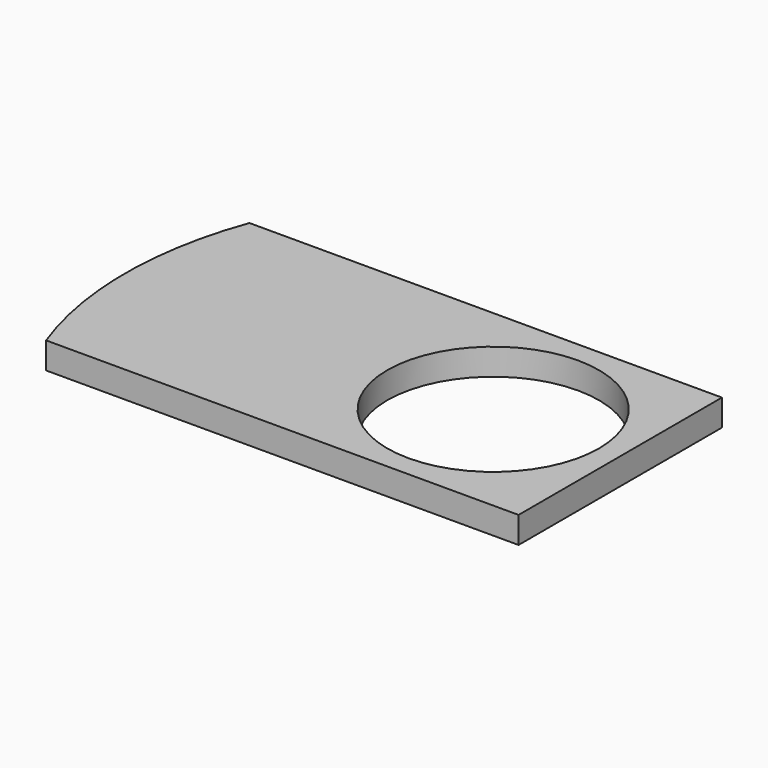
from build123d import *

# Parameters (mm, degrees)
F0_R     = 2
F1_DEPTH = 0.5


with BuildPart() as f1:
    # F0 (on Top) → F1 (new body)
    with BuildSketch(Plane.XY):
        with BuildLine():
            Line((-5.986860613, 2.4), (-6.5224611919, 2.4))
            ThreePointArc((-6.5224611919, 2.4), (-6.95, 0), (-6.5224611919, -2.4))
            Line((-6.5224611919, -2.4), (-5.986860613, -2.4))
            ThreePointArc((-5.986860613, -2.4), (-6.45, 0), (-5.986860613, 2.4))
        make_face()
        with BuildLine():
            Line((2.4, -2.4), (2.4, 2.4))
            Line((2.4, 2.4), (-5.986860613, 2.4))
            ThreePointArc((-5.986860613, 2.4), (-6.45, 0), (-5.986860613, -2.4))
            Line((-5.986860613, -2.4), (2.4, -2.4))
        make_face()
        Circle(F0_R, mode=Mode.SUBTRACT)
    extrude(amount=F1_DEPTH)


solid = f1.part
